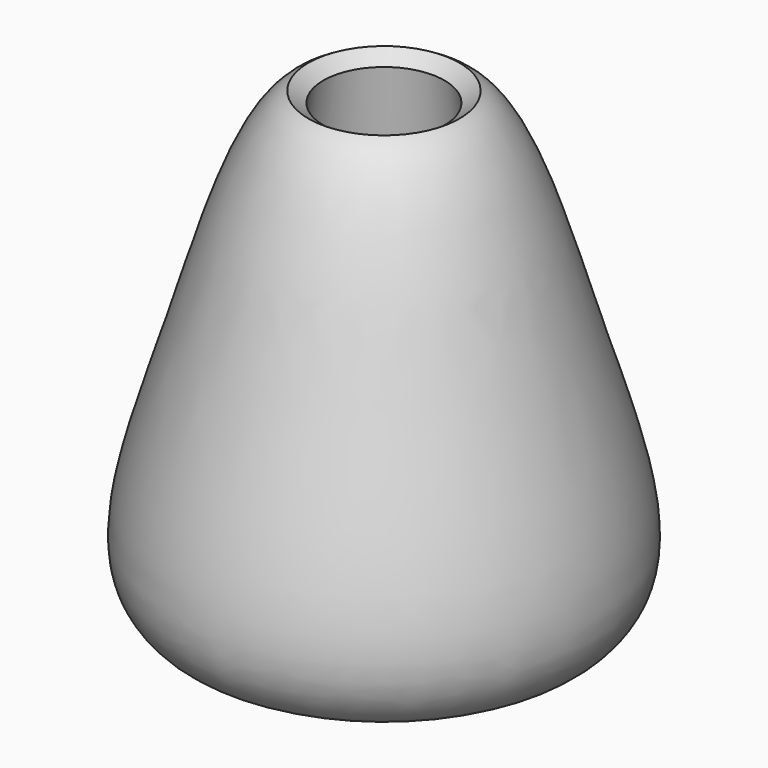
from build123d import *


# Not quite as in the source:
# - a fillet or chamfer that OpenCascade refuses, or shapes differently, is made with other operations: its cross-section is extruded or revolved along the edge and cut away or added


with BuildPart() as f1:
    # F0 (on Front) → F1 (revolve)
    with BuildSketch(Plane.XZ):
        with BuildLine():
            Line((-3.5, 0), (-2.5, 0))
            Line((-2.5, 0), (-1.25, 10))
            add(Edge.make_bspline(
                [(-3.5, 0), (-3.9109399026, 0), (-5.1379781007, 1.1218116101), (-3.583476839, 5.2947134956), (-2.3579561905, 10.0052182198), (-1.25, 10)],
                knots=[0, 0, 0, 0, 0.2111554637, 0.5999875956, 1, 1, 1, 1], degree=3))
        make_face()
    revolve(axis=Axis((0, 0, 5), (0, 0, 1)))

    # F2: chamfer of 0.25 on 1 edges, made by hand

    # F2_s1 → F2_t2 (revolve, cut)
    with BuildSketch(Plane.XZ):
        with BuildLine():
            Line((-1.2808466604, 9.6821580362), (-1.6162215087, 9.9196286061))
            Line((-1.6162215087, 9.9196286061), (-1.6184542391, 9.9241024093))
            ThreePointArc((-1.6184542391, 9.9241024093), (-1.4387043558, 9.9822574227), (-1.2499764514, 10.0049999445))
            Line((-1.2499764514, 10.0049999445), (-1.2450386106, 9.9993798263))
            ThreePointArc((-1.2450386106, 9.9993798263), (-1.2648353981, 9.8410055266), (-1.275885271, 9.6815378625))
            Line((-1.275885271, 9.6815378625), (-1.2808466604, 9.6821580362))
        make_face()
    revolve(axis=Axis((0, 0, 10), (0, 0, 1)), mode=Mode.SUBTRACT)


solid = f1.part
